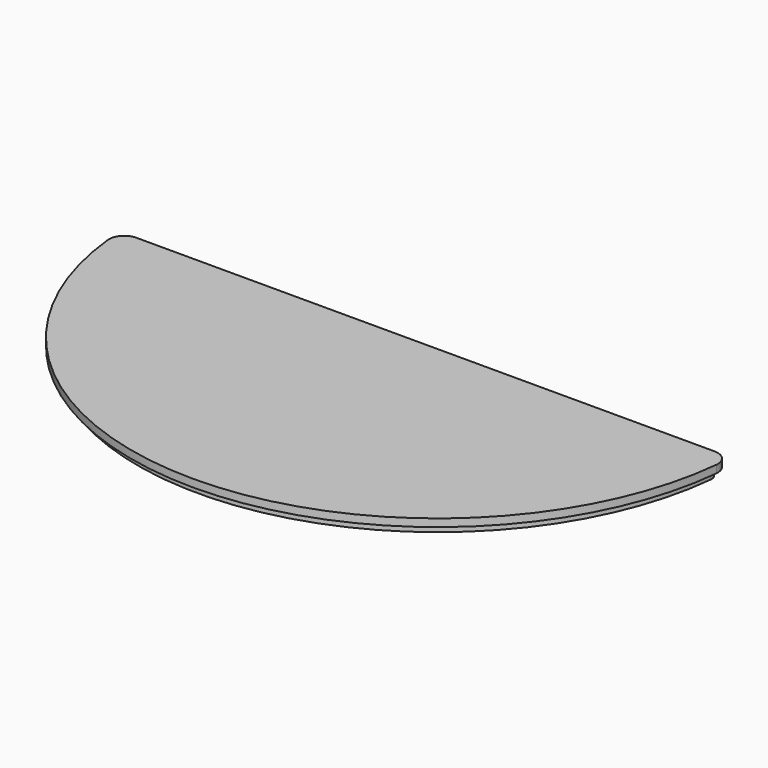
from build123d import *

# Parameters (mm, degrees)
F1_DEPTH = 1
F2_DEPTH = 1


with BuildPart() as f1:
    # F0 (on Top) → F1 (new body)
    with BuildSketch(Plane.XY):
        with BuildLine():
            ThreePointArc((28.507673021, -4.2105263158), (28.0055681014, -2.6622878919), (26.5187842181, -2))
            Line((26.5187842181, -2), (-49.0589902927, -2))
            ThreePointArc((-49.0589902927, -2), (-50.5457741761, -2.6622878919), (-51.0478790956, -4.2105263158))
            ThreePointArc((-51.0478790956, -4.2105263158), (-11.2701030373, -40), (28.507673021, -4.2105263158))
        make_face()
        with BuildLine():
            ThreePointArc((26.5187842181, -2.7999999982), (27.4108545494, -3.1973727339), (27.7121175016, -4.1263157897))
            ThreePointArc((27.7121175016, -4.1263157897), (-11.2701030383, -39.2000000018), (-50.2523235764, -4.1263157876))
            ThreePointArc((-50.2523235764, -4.1263157876), (-49.9510606247, -3.1973727333), (-49.0589902947, -2.7999999982))
            Line((-49.0589902947, -2.7999999982), (26.5187842181, -2.7999999982))
        make_face(mode=Mode.SUBTRACT)
        with BuildLine():
            ThreePointArc((-50.2523235764, -4.1263157876), (-11.2701030383, -39.2000000018), (27.7121175016, -4.1263157897))
            ThreePointArc((27.7121175016, -4.1263157897), (27.4108545494, -3.1973727339), (26.5187842181, -2.7999999982))
            Line((26.5187842181, -2.7999999982), (-49.0589902947, -2.7999999982))
            ThreePointArc((-49.0589902947, -2.7999999982), (-49.9510606247, -3.1973727333), (-50.2523235764, -4.1263157876))
        make_face()
        with BuildLine():
            Line((-49.0589902947, -3.5999999382), (26.5187842181, -3.5999999382))
            ThreePointArc((26.5187842181, -3.5999999382), (26.8161410407, -3.732457537), (26.9165620401, -4.0421052697))
            ThreePointArc((26.9165620401, -4.0421052697), (-11.2701030383, -38.4000000618), (-49.456768115, -4.0421052677))
            ThreePointArc((-49.456768115, -4.0421052677), (-49.356347116, -3.7324575364), (-49.0589902947, -3.5999999382))
        make_face(mode=Mode.SUBTRACT)
        with BuildLine():
            ThreePointArc((26.9165620401, -4.0421052697), (26.8161410407, -3.732457537), (26.5187842181, -3.5999999382))
            Line((26.5187842181, -3.5999999382), (-49.0589902947, -3.5999999382))
            ThreePointArc((-49.0589902947, -3.5999999382), (-49.356347116, -3.7324575364), (-49.456768115, -4.0421052677))
            ThreePointArc((-49.456768115, -4.0421052677), (-11.2701030383, -38.4000000618), (26.9165620401, -4.0421052697))
        make_face()
    extrude(amount=F1_DEPTH)

    # F0 (on Top) → F2 (join)
    with BuildSketch(Plane.XY):
        with BuildLine():
            ThreePointArc((-50.2523235764, -4.1263157876), (-11.2701030383, -39.2000000018), (27.7121175016, -4.1263157897))
            ThreePointArc((27.7121175016, -4.1263157897), (27.4108545494, -3.1973727339), (26.5187842181, -2.7999999982))
            Line((26.5187842181, -2.7999999982), (-49.0589902947, -2.7999999982))
            ThreePointArc((-49.0589902947, -2.7999999982), (-49.9510606247, -3.1973727333), (-50.2523235764, -4.1263157876))
        make_face()
        with BuildLine():
            Line((-49.0589902947, -3.5999999382), (26.5187842181, -3.5999999382))
            ThreePointArc((26.5187842181, -3.5999999382), (26.8161410407, -3.732457537), (26.9165620401, -4.0421052697))
            ThreePointArc((26.9165620401, -4.0421052697), (-11.2701030383, -38.4000000618), (-49.456768115, -4.0421052677))
            ThreePointArc((-49.456768115, -4.0421052677), (-49.356347116, -3.7324575364), (-49.0589902947, -3.5999999382))
        make_face(mode=Mode.SUBTRACT)
    extrude(amount=-F2_DEPTH)


solid = f1.part
